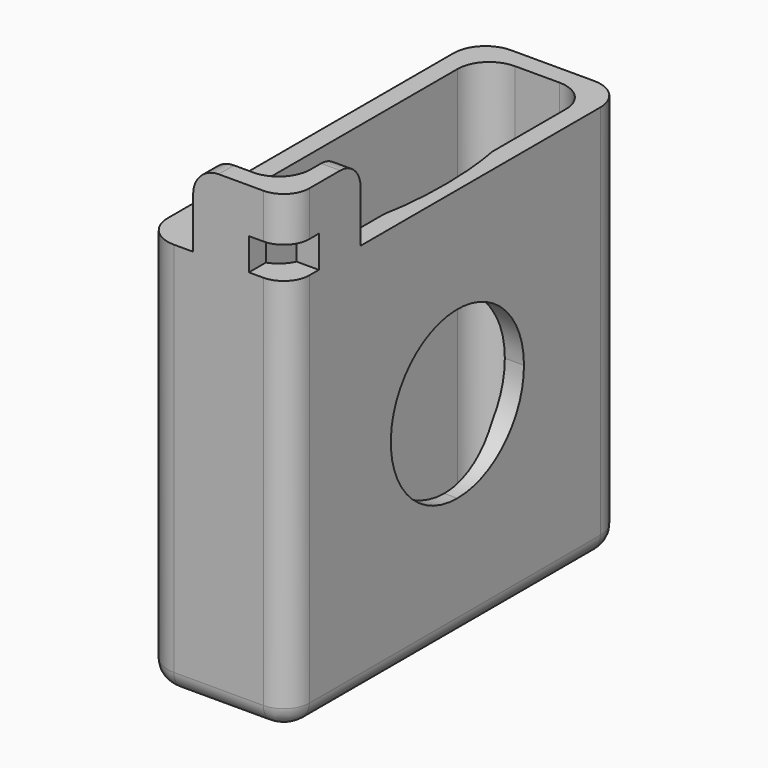
from build123d import *

# Parameters (mm, degrees)
F0_W         = 2.23
F0_H         = 8.65
F1_DEPTH     = 1.5
F2_DEPTH     = 31
F5_DEPTH     = 2
F6_R         = 1.5
F7_DEPTH     = 6
F8_R         = 2
F9_DEPTH     = 2.5
F10_T1_DEPTH = 13.5
F10_T3_DEPTH = 36
F10_T6_ANGLE = 90


# Not quite as in the source:
# - a fillet or chamfer that OpenCascade refuses, or shapes differently, is made with other operations: its cross-section is extruded or revolved along the edge and cut away or added
# - a feature names something its author has since deleted; it is built from what else it names


with BuildPart() as f1:
    # F0 (on Top) → F1 (new body)
    with BuildSketch(Plane.XY):
        with BuildLine():
            Line((-1.75, -15), (1.75, -15))
            ThreePointArc((1.75, -15), (3.517766953, -14.267766953), (4.25, -12.5))
            Line((4.25, -12.5), (4.25, -5.3126580607))
            add(Edge.make_bspline(
                [(4.25, -5.3126580607), (5.242489647, 0), (4.25, 5.3126580607)],
                knots=[4.2622339472, 4.2622339472, 4.2622339472, 5.1625440136, 5.1625440136, 5.1625440136], degree=2, weights=[1, 0.9003796574, 1]))
            Line((4.25, 5.3126580607), (4.25, 12.5))
            ThreePointArc((4.25, 12.5), (3.517766953, 14.267766953), (1.75, 15))
            Line((1.75, 15), (-1.75, 15))
            ThreePointArc((-1.75, 15), (-3.517766953, 14.267766953), (-4.25, 12.5))
            Line((-4.25, 12.5), (-4.25, -12.5))
            ThreePointArc((-4.25, -12.5), (-3.517766953, -14.267766953), (-1.75, -15))
        make_face()
        Rectangle(F0_W, F0_H, mode=Mode.SUBTRACT)
    extrude(amount=F1_DEPTH)

    # F0 (on Top) → F2 (join)
    with BuildSketch(Plane.XY):
        with BuildLine():
            ThreePointArc((5.75, 14), (5.017766953, 15.767766953), (3.25, 16.5))
            Line((3.25, 16.5), (-3.25, 16.5))
            ThreePointArc((-3.25, 16.5), (-5.017766953, 15.767766953), (-5.75, 14))
            Line((-5.75, 14), (-5.75, -14))
            ThreePointArc((-5.75, -14), (-5.017766953, -15.767766953), (-3.25, -16.5))
            Line((-3.25, -16.5), (5.75, -16.5))
            Line((5.75, -16.5), (5.75, 14))
        make_face()
        with BuildLine():
            ThreePointArc((4.25, -12.5), (3.517766953, -14.267766953), (1.75, -15))
            Line((1.75, -15), (-1.75, -15))
            ThreePointArc((-1.75, -15), (-3.517766953, -14.267766953), (-4.25, -12.5))
            Line((-4.25, -12.5), (-4.25, 12.5))
            ThreePointArc((-4.25, 12.5), (-3.517766953, 14.267766953), (-1.75, 15))
            Line((-1.75, 15), (1.75, 15))
            ThreePointArc((1.75, 15), (3.517766953, 14.267766953), (4.25, 12.5))
            Line((4.25, 12.5), (4.25, 5.3126580607))
            add(Edge.make_bspline(
                [(4.25, -5.3126580607), (5.242489647, 0), (4.25, 5.3126580607)],
                knots=[4.2622339472, 4.2622339472, 4.2622339472, 5.1625440136, 5.1625440136, 5.1625440136], degree=2, weights=[1, 0.9003796574, 1]))
            Line((4.25, -5.3126580607), (4.25, -12.5))
        make_face(mode=Mode.SUBTRACT)
    extrude(amount=F2_DEPTH)

    # F4 (on face) → F5 (cut)
    with BuildSketch(Plane.YZ.offset(5.75)):
        with BuildLine():
            ThreePointArc((6.52, 16.25), (-4.6103362133, 20.8603362133), (0, 9.73))
            ThreePointArc((0, 9.73), (4.6103362133, 11.6396637867), (6.52, 16.25))
        make_face()
    extrude(amount=-F5_DEPTH, mode=Mode.SUBTRACT)

    # F6
    f6_edges = [f1.edges().sort_by_distance(p)[0] for p in [
        (5.75, -1.25, 0),
    ]]
    fillet(f6_edges, radius=F6_R)

    # F3 (on face) → F7 (join)
    with BuildSketch(Plane.XY.offset(31)):
        with BuildLine():
            Line((2.6164813973, -14.8450394427), (2.6164813973, -16.5))
            Line((2.6164813973, -16.5), (5.75, -16.5))
            Line((5.75, -16.5), (5.75, -13.5683528888))
            Line((5.75, -13.5683528888), (4.0102261181, -13.5683528888))
            ThreePointArc((4.0102261181, -13.5683528888), (3.4386554151, -14.3434866121), (2.6164813973, -14.8450394427))
        make_face()
        with BuildLine():
            Line((4.0102261181, -13.5683528888), (5.75, -13.5683528888))
            Line((5.75, -13.5683528888), (5.75, -9.473525919))
            Line((5.75, -9.473525919), (4.25, -9.473525919))
            Line((4.25, -9.473525919), (4.25, -12.5))
            ThreePointArc((4.25, -12.5), (4.18932012, -13.0474644759), (4.0102261181, -13.5683528888))
        make_face()
        with BuildLine():
            Line((-1.75, -15), (-1.75, -16.5))
            Line((-1.75, -16.5), (2.6164813973, -16.5))
            Line((2.6164813973, -16.5), (2.6164813973, -14.8450394427))
            ThreePointArc((2.6164813973, -14.8450394427), (2.190114413, -14.9609549576), (1.75, -15))
            Line((1.75, -15), (-1.75, -15))
        make_face()
    extrude(amount=F7_DEPTH)

    # F8
    f8_edges = [f1.edges().sort_by_distance(p)[0] for p in [
        (-1.75, -15.75, 37),
        (5, -9.473526, 37),
    ]]
    fillet(f8_edges, radius=F8_R)

    # F3 (on face) → F9 (cut)
    with BuildSketch(Plane.XY.offset(31)):
        with BuildLine():
            Line((2.6164813973, -14.8450394427), (2.6164813973, -16.5))
            Line((2.6164813973, -16.5), (5.75, -16.5))
            Line((5.75, -16.5), (5.75, -13.5683528888))
            Line((5.75, -13.5683528888), (4.0102261181, -13.5683528888))
            ThreePointArc((4.0102261181, -13.5683528888), (3.4386554151, -14.3434866121), (2.6164813973, -14.8450394427))
        make_face()
    extrude(amount=F9_DEPTH, mode=Mode.SUBTRACT)

    # F10: fillet of radius 2 on 2 edges, made by hand

    # F10_s2 → F10_t1 (cut)
    with BuildSketch(Plane.XY.offset(28.5)):
        with BuildLine():
            ThreePointArc((5.75, -14.5), (5.1642135624, -15.9142135624), (3.75, -16.5))
            Line((3.75, -16.5), (5.75, -16.5))
            Line((5.75, -16.5), (5.75, -14.5))
        make_face()
    extrude(amount=F10_T1_DEPTH, mode=Mode.SUBTRACT)

    # F10_s4 → F10_t3 (cut)
    with BuildSketch(Plane.XY):
        with BuildLine():
            ThreePointArc((5.75, -14.5), (5.1642135624, -15.9142135624), (3.75, -16.5))
            Line((3.75, -16.5), (5.75, -16.5))
            Line((5.75, -16.5), (5.75, -14.5))
        make_face()
    extrude(amount=F10_T3_DEPTH, mode=Mode.SUBTRACT)

    # F10_s5 → F10_t6 (revolve, cut)
    with BuildSketch(Plane.XZ.offset(14.5)):
        with BuildLine():
            ThreePointArc((4.25, 0), (5.3106601718, 0.4393398282), (5.75, 1.5))
            Line((5.75, 1.5), (5.75, 0))
            Line((5.75, 0), (4.25, 0))
        make_face()
    revolve(axis=Axis((3.75, -14.5, 0), (0, 0, -1)), revolution_arc=F10_T6_ANGLE, mode=Mode.SUBTRACT)


solid = f1.part
